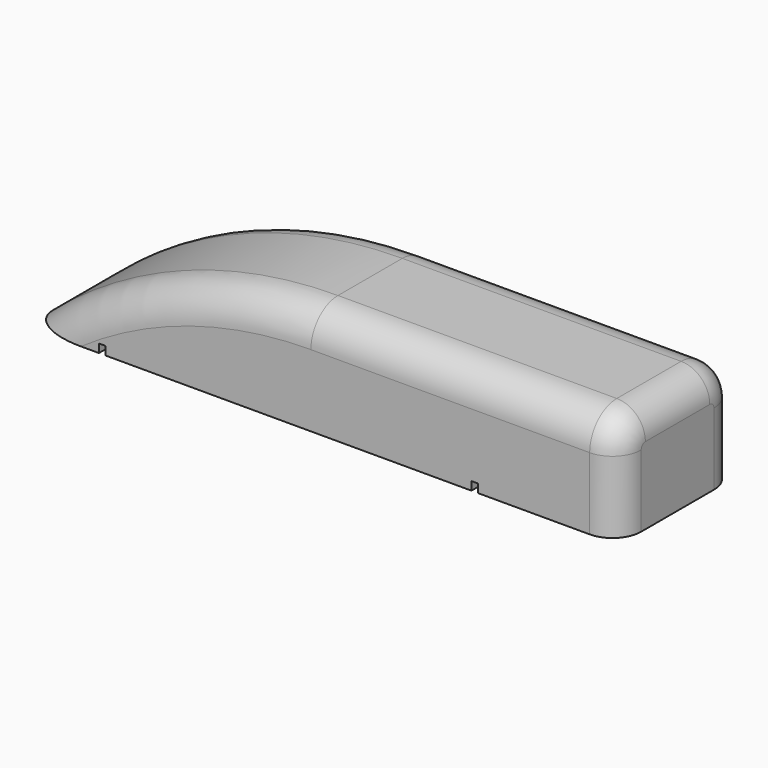
from build123d import *

# Parameters (mm, degrees)
F0_W        = 177.8
F0_H        = 44.45
F1_DEPTH    = 31.75
F2_W        = 2.032
F2_H        = 5.08
F2_H_2      = 2.957622528
F3_DEPTH    = 70.866
F4_T1_DEPTH = 472.3767319638
F5_R        = 10.16
F6_R        = 10.16
F7_R        = 8.5849434278
F8_W        = 78.1799629331
F8_H        = 27.9869418591
F9_DEPTH    = 12.7


# Not quite as in the source:
# - a fillet or chamfer that OpenCascade refuses, or shapes differently, is made with other operations: its cross-section is extruded or revolved along the edge and cut away or added


with BuildPart() as f1:
    # F0 (on Top) → F1 (new body)
    with BuildSketch(Plane.XY):
        Rectangle(F0_W, F0_H)
    extrude(amount=F1_DEPTH)

    # F2 (on Front) → F3 (cut, symmetric)
    with BuildSketch(Plane.XZ):
        with Locations((-65.8876, 0)):
            Rectangle(F2_W, F2_H)
        with Locations((45.8724, 1.061188736)):
            Rectangle(F2_W, F2_H_2)
    extrude(amount=F3_DEPTH, both=True, mode=Mode.SUBTRACT)

    # F4: fillet of radius 131.2269923964 on 1 edges, made by hand

    # F4_s2 → F4_t1 (cut)
    with BuildSketch(Plane.XZ.offset(-236.1883659819)):
        with BuildLine():
            ThreePointArc((-3.3146536072, 31.75), (-48.9570517069, 23.5567226134), (-88.9, 0))
            Line((-88.9, 0), (-88.9, 31.75))
            Line((-88.9, 31.75), (-3.3146536072, 31.75))
        make_face()
    extrude(amount=F4_T1_DEPTH, mode=Mode.SUBTRACT)

    # F5
    f5_edges = [f1.edges().sort_by_distance(p)[0] for p in [
        (-48.957052, -22.225, 23.556723),
    ]]
    fillet(f5_edges, radius=F5_R)

    # F6
    f6_edges = [f1.edges().sort_by_distance(p)[0] for p in [
        (42.792673, 22.225, 31.75),
        (-48.957052, 22.225, 23.556723),
    ]]
    fillet(f6_edges, radius=F6_R)

    # F7
    f7_edges = [f1.edges().sort_by_distance(p)[0] for p in [
        (88.9, 0, 31.75),
        (88.9, 22.225, 10.795),
        (88.9, -22.225, 10.795),
        (88.9, 19.249205, 28.774205),
        (88.9, -19.249205, 28.774205),
    ]]
    fillet(f7_edges, radius=F7_R)

    # F8 (on Top) → F9 (cut, symmetric)
    with BuildSketch(Plane.XY):
        Rectangle(F8_W, F8_H)
    extrude(amount=F9_DEPTH, both=True, mode=Mode.SUBTRACT)


solid = f1.part
